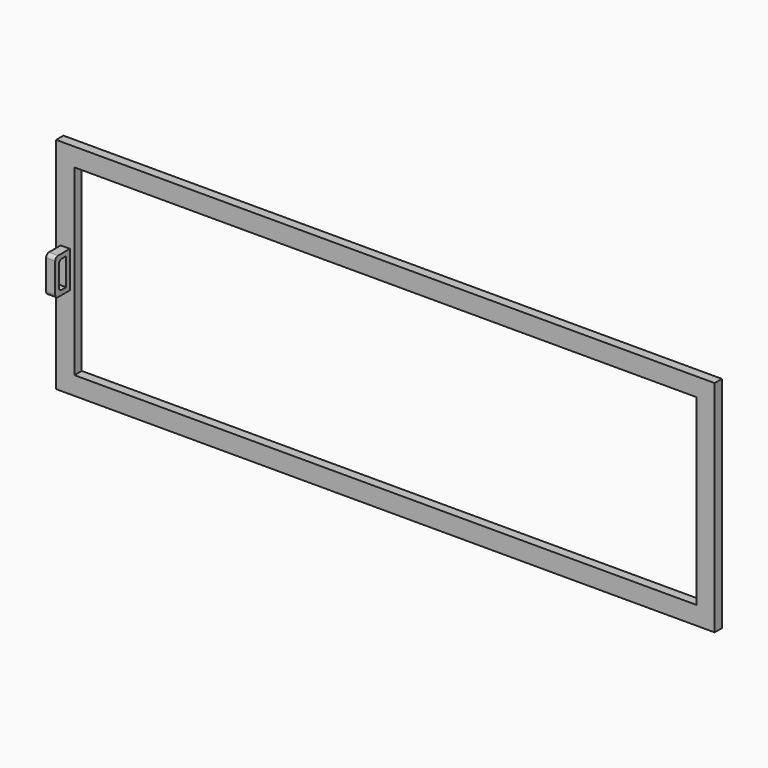
from build123d import *

# Parameters (mm, degrees)
F0_W     = 914.4
F0_H     = 304.8
F0_W_2   = 863.6
F0_H_2   = 254
F1_DEPTH = 6.35
F3_DEPTH = 25.4
F5_DEPTH = 25.4
F6_R     = 5.08
F7_R     = 5.08


with BuildPart() as f1:
    # F0 (on Front) → F1 (new body, symmetric)
    with BuildSketch(Plane.XZ):
        Rectangle(F0_W, F0_H)
        Rectangle(F0_W_2, F0_H_2, mode=Mode.SUBTRACT)
    extrude(amount=F1_DEPTH, both=True)

    # F2 (on face) → F3 (join)
    with BuildSketch(Plane.XZ.offset(6.35)):
        Polygon((-438.15, 0), (-438.15, 25.4), (-450.85, 25.4), (-450.85, -25.4), (-438.15, -25.4), align=None)
    extrude(amount=F3_DEPTH)

    # F4 (on face) → F5 (cut)
    with BuildSketch(Plane(origin=(-450.85, 0, 0), x_dir=(0, -1, 0), z_dir=(-1, 0, 0))):
        Polygon((25.4, 0), (25.4, 19.05), (12.7, 19.05), (12.7, -19.05), (25.4, -19.05), align=None)
    extrude(amount=-F5_DEPTH, mode=Mode.SUBTRACT)

    # F6
    f6_edges = [f1.edges().sort_by_distance(p)[0] for p in [
        (-444.5, -25.4, 19.05),
        (-444.5, -25.4, -19.05),
    ]]
    fillet(f6_edges, radius=F6_R)

    # F7
    f7_edges = [f1.edges().sort_by_distance(p)[0] for p in [
        (-444.5, -31.75, 25.4),
        (-444.5, -31.75, -25.4),
    ]]
    fillet(f7_edges, radius=F7_R)


solid = f1.part
